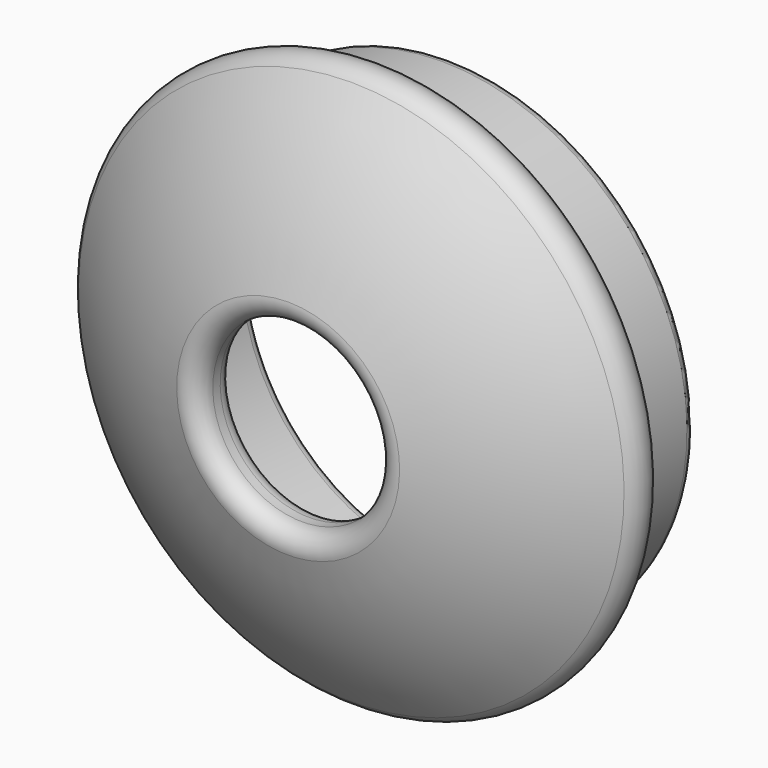
from build123d import *


# Not quite as in the source:
# - ends of sketch curves that miss each other by under 0.0002 mm in the source are joined


with BuildPart() as f1:
    # F0 (on Right) → F1 (revolve)
    with BuildSketch(Plane.YZ):
        with BuildLine():
            ThreePointArc((-2.0831162887, 2.5), (-2.0120457201, 2.1550510257), (-1.6958179541, 2))
            Line((-1.6958179541, 2), (-1.4891121437, 2))
            ThreePointArc((-1.4891121437, 2), (-1.2450333284, 2.0831001232), (-1.1023694112, 2.2978723405))
            ThreePointArc((-1.1023694112, 2.2978723405), (-0.7217967722, 3.4290885624), (-0.1948865645, 4.5))
            ThreePointArc((-0.1948865645, 4.5), (0.1235230232, 5.0112004142), (0.475408639, 5.4999611351))
            ThreePointArc((0.475408639, 5.4999611351), (0.4777809564, 5.5030325568), (0.4801545979, 5.5061029552))
            ThreePointArc((0.4801545979, 5.5061029552), (0.5801024047, 5.8792370625), (0.3843238308, 6.2122376272))
            ThreePointArc((0.3843238358, 6.2122376234), (0.0174046888, 6.3074557819), (-0.3108662275, 6.1178921683))
            ThreePointArc((-0.3108662275, 6.1178921683), (-1.3810680516, 4.3991174031), (-2.0831162887, 2.5))
        make_face()
        with BuildLine():
            ThreePointArc((0.475408639, 5.4999611351), (0.1235230232, 5.0112004142), (-0.1948865645, 4.5))
            Line((-0.1948865645, 4.5), (2.2253582985, 4.5))
            ThreePointArc((2.2253582985, 4.5), (2.4021349938, 4.5732233047), (2.4753582985, 4.75))
            Line((2.4753582985, 4.75), (2.4753582985, 5.25))
            ThreePointArc((2.4753582985, 5.25), (2.4021349938, 5.4267766953), (2.2253582985, 5.5))
            Line((2.2253582985, 5.5), (0.475408639, 5.4999611351))
        make_face()
    revolve(axis=Axis((0, -2.938644262, 0), (0, -1, 0)))


solid = f1.part
